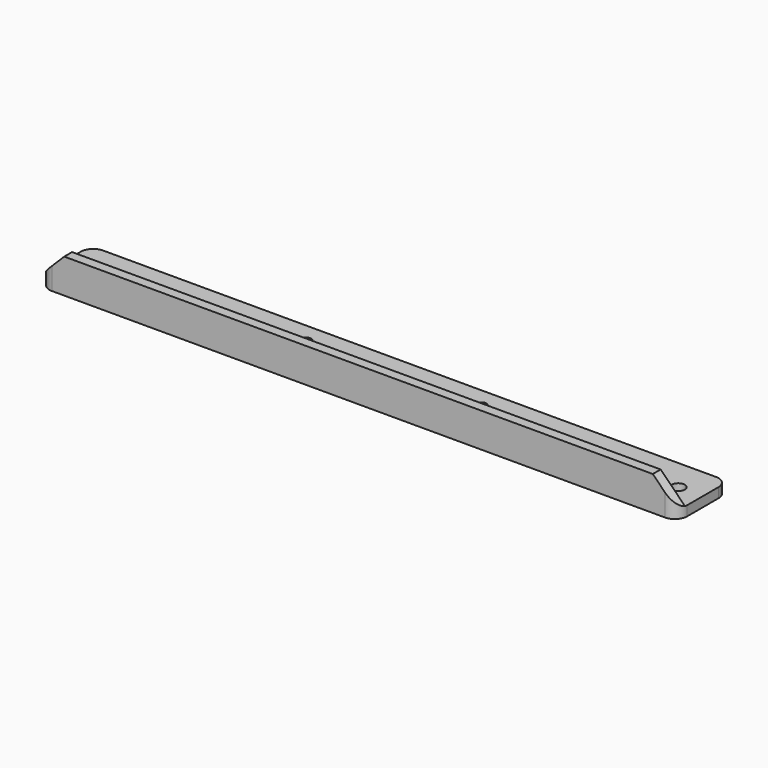
from build123d import *

# Parameters (mm, degrees)
F0_W        = 260
F0_H        = 26
F0_R        = 2.7
F0_R_2      = 2
F1_DEPTH    = 4
F2_W        = 260
F2_H        = 4
F3_DEPTH    = 10
F4_SIZE     = 10
F5_T1_DEPTH = 29


# Not quite as in the source:
# - a fillet or chamfer that OpenCascade refuses, or shapes differently, is made with other operations: its cross-section is extruded or revolved along the edge and cut away or added


with BuildPart() as f1:
    # F0 (on Top) → F1 (new body)
    with BuildSketch(Plane.XY):
        Rectangle(F0_W, F0_H)
        with Locations((-120, 0)):
            Circle(F0_R, mode=Mode.SUBTRACT)
        with Locations((-35.75, 5)):
            Circle(F0_R_2, mode=Mode.SUBTRACT)
        with Locations((35.75, 5)):
            Circle(F0_R_2, mode=Mode.SUBTRACT)
        with Locations((120, 0)):
            Circle(F0_R, mode=Mode.SUBTRACT)
    extrude(amount=F1_DEPTH)

    # F2 (on face) → F3 (join)
    with BuildSketch(Plane.XY.offset(4)):
        with Locations((0, -11)):
            Rectangle(F2_W, F2_H)
    extrude(amount=F3_DEPTH)

    # F4
    f4_edges = [f1.edges().sort_by_distance(p)[0] for p in [
        (-130, -11, 14),
        (130, -11, 14),
    ]]
    chamfer(f4_edges, length=F4_SIZE)

    # F5: fillet of radius 5 on 4 edges, made by hand

    # F5_s2 → F5_t1 (cut)
    with BuildSketch(Plane.XY.offset(-12.5)):
        with BuildLine():
            ThreePointArc((125, 13), (128.5355339059, 11.5355339059), (130, 8))
            Line((130, 8), (130, 13))
            Line((130, 13), (125, 13))
        make_face()
        with BuildLine():
            ThreePointArc((125, -13), (128.5355339059, -11.5355339059), (130, -8))
            Line((130, -8), (130, -13))
            Line((130, -13), (125, -13))
        make_face()
        with BuildLine():
            ThreePointArc((-130, 8), (-128.5355339059, 11.5355339059), (-125, 13))
            Line((-125, 13), (-130, 13))
            Line((-130, 13), (-130, 8))
        make_face()
        with BuildLine():
            ThreePointArc((-130, -8), (-128.5355339059, -11.5355339059), (-125, -13))
            Line((-125, -13), (-130, -13))
            Line((-130, -13), (-130, -8))
        make_face()
    extrude(amount=F5_T1_DEPTH, mode=Mode.SUBTRACT)


solid = f1.part
